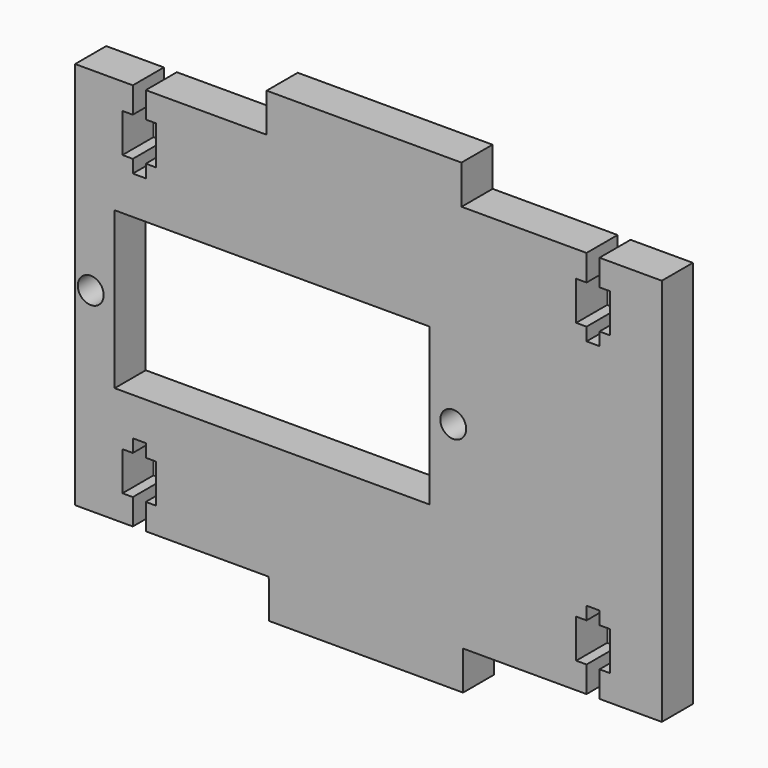
from build123d import *

# Parameters (mm, degrees)
F3_W     = 24.3006017764
F3_H     = 12.100000065
F3_R     = 1
F4_DEPTH = 3


# Not quite as in the source:
# - ends of sketch curves that miss each other by under 0.0002 mm in the source are joined


with BuildPart() as f4:
    # F3 (on Front) → F4 (new body)
    with BuildSketch(Plane.XZ):
        Polygon((-18.3427034128, 0), (-17.3427034128, 0), (-17.3423305717, 1.9999998262), (-18.1417713099, 1.9999998262), (-18.1417713099, 4.9999998262), (-17.3417713099, 4.9999998262), (-17.3415848893, 5.9999998262), (-16.3415848684, 5.9999998262), (-16.3417712925, 4.9999998262), (-15.5417712925, 4.9999998262), (-15.5417712925, 1.9999998262), (-16.3423305647, 1.9999998262), (-16.3427034128, 0), (-15.3427034128, 0), (-6.8427034128, 0), (8.1310835591, 0), (8.1572965872, 0), (16.6572965872, 0), (17.7038592511, 0), (17.704234553, 2.0131421474), (16.9047938148, 2.0131421517), (16.9047938308, 5.0131421517), (17.7047938308, 5.0131421475), (17.7049802567, 6.0131421474), (18.7049802776, 6.0131421421), (18.7047938482, 5.0131421421), (19.5047938482, 5.0131421378), (19.5047938321, 2.0131421378), (18.7042345599, 2.0131421421), (18.703859251, 0), (19.6572965872, 0), (23.5180836171, 0), (23.5180836171, 30), (18.7038593313, 30), (18.7042346294, 27.9868579887), (19.5047939016, 27.9868579887), (19.5047939016, 24.9868579887), (18.7047939016, 24.9868579887), (18.7049803257, 23.9868579887), (17.7049803048, 23.9868579887), (17.7047938842, 24.9868579887), (16.9047938842, 24.9868579887), (16.9047938842, 27.9868579887), (17.7042346225, 27.9868579887), (17.7038593313, 30), (8.0515714362, 30), (0, 30), (-7.0037143305, 30), (-16.3427034128, 30), (-16.3423305647, 28.0000001738), (-15.5417712925, 28.0000001738), (-15.5417712925, 25.0000001738), (-16.3417712925, 25.0000001738), (-16.3415848684, 24.0000001738), (-17.3415848893, 24.0000001738), (-17.3417713099, 25.0000001738), (-18.1417713099, 25.0000001738), (-18.1417713099, 28.0000001738), (-17.3423305717, 28.0000001738), (-17.3427034128, 30), (-21.7979144805, 30), (-21.7979144805, 28.0000001738), (-21.7979144805, 25.0000001738), (-21.7979144805, 24.0000001738), (-21.7979144805, 15.0000001738), (-21.7979144805, 1.738e-07), align=None)
        with BuildLine():
            ThreePointArc((-19.593004301, 15.0000001705), (-20.5930043024, 14.0000001705), (-21.593004301, 15.0000001732))
            ThreePointArc((-21.593004301, 15.0000001732), (-20.5930042997, 16.0000001705), (-19.593004301, 15.0000001705))
        make_face(mode=Mode.SUBTRACT)
        with Locations((-6.593004301, 15.0000001331)):
            Rectangle(F3_W, F3_H, mode=Mode.SUBTRACT)
        with Locations((7.406995699, 15.0000000956)):
            Circle(F3_R, mode=Mode.SUBTRACT)
        Polygon((-7.0037143305, 33), (-7.0037143305, 30), (0, 30), (8.0515714362, 30), (8.0409989211, 33), align=None)
        Polygon((8.1310835591, 0), (-6.8427034128, 0), (-6.826602321, -3), (0, -3), (8.1678691023, -3), (8.1572965872, 0), align=None)
    extrude(amount=F4_DEPTH)


solid = f4.part
